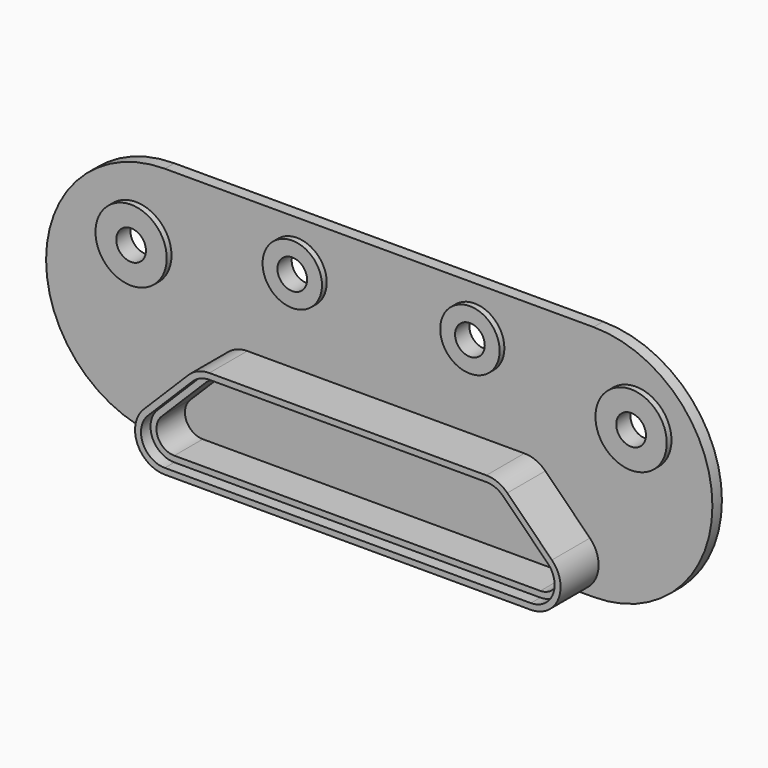
from build123d import *

# Parameters (mm, degrees)
F1_DEPTH  = 2
F3_DEPTH  = 8
F5_DEPTH  = 2
F7_DEPTH  = 6
F8_R      = 5
F8_R_2    = 6
F9_DEPTH  = 1
F10_R     = 2.5
F11_R     = 2.5
F12_DEPTH = 3.001


# Not quite as in the source:
# - a feature names something its author has since deleted; it is built from what else it names


with BuildPart() as f1:
    # F0 (on Front) → F1 (new body)
    with BuildSketch(Plane.XZ):
        with BuildLine():
            Line((-37.1916021632, -20), (34.9713978368, -20))
            ThreePointArc((34.9713978368, -20), (54.9713978368, 0), (34.9713978368, 20))
            Line((34.9713978368, 20), (-37.1916021632, 20))
            ThreePointArc((-37.1916021632, 20), (-57.1916021632, 0), (-37.1916021632, -20))
        make_face()
    extrude(amount=F1_DEPTH)

    # F2 (on face) → F3 (join)
    with BuildSketch(Plane.XZ.offset(2)):
        with BuildLine():
            Line((23.3145, -2.5), (0, -2.5))
            Line((0, -2.5), (-23.3145, -2.5))
            ThreePointArc((-23.3145, -2.5), (-25.2279171618, -2.8806023374), (-26.8500339059, -3.9644660941))
            Line((-26.8500339059, -3.9644660941), (-34.3500339059, -11.4644660941))
            ThreePointArc((-34.3500339059, -11.4644660941), (-35.4338976626, -16.9134171618), (-30.8145, -20))
            Line((-30.8145, -20), (0, -20))
            Line((0, -20), (30.8145, -20))
            ThreePointArc((30.8145, -20), (35.4338976626, -16.9134171618), (34.3500339059, -11.4644660941))
            Line((34.3500339059, -11.4644660941), (26.8500339059, -3.9644660941))
            ThreePointArc((26.8500339059, -3.9644660941), (25.2279171618, -2.8806023374), (23.3145, -2.5))
        make_face()
    extrude(amount=F3_DEPTH)

    # F4 (on face) → F5 (cut)
    with BuildSketch(Plane.XZ.offset(10)):
        with BuildLine():
            Line((-26.1429271247, -4.6715728753), (-33.6429271247, -12.1715728753))
            ThreePointArc((-33.6429271247, -12.1715728753), (-34.51001813, -16.5307337295), (-30.8145, -19))
            Line((-30.8145, -19), (30.8145, -19))
            ThreePointArc((30.8145, -19), (34.51001813, -16.5307337295), (33.6429271247, -12.1715728753))
            Line((33.6429271247, -12.1715728753), (26.1429271247, -4.6715728753))
            ThreePointArc((26.1429271247, -4.6715728753), (24.8452337295, -3.80448187), (23.3145, -3.5))
            Line((23.3145, -3.5), (-23.3145, -3.5))
            ThreePointArc((-23.3145, -3.5), (-24.8452337295, -3.80448187), (-26.1429271247, -4.6715728753))
        make_face()
    extrude(amount=-F5_DEPTH, mode=Mode.SUBTRACT)

    # F6 (on face) → F7 (cut)
    with BuildSketch(Plane.XZ.offset(8)):
        with BuildLine():
            ThreePointArc((30.8145, -18), (33.5861385975, -16.1480502971), (32.9358203436, -12.8786796564))
            Line((32.9358203436, -12.8786796564), (25.4358203436, -5.3786796564))
            ThreePointArc((25.4358203436, -5.3786796564), (24.4625502971, -4.7283614025), (23.3145, -4.5))
            Line((23.3145, -4.5), (-23.3145, -4.5))
            ThreePointArc((-23.3145, -4.5), (-24.4625502971, -4.7283614025), (-25.4358203436, -5.3786796564))
            Line((-25.4358203436, -5.3786796564), (-32.9358203436, -12.8786796564))
            ThreePointArc((-32.9358203436, -12.8786796564), (-33.5861385975, -16.1480502971), (-30.8145, -18))
            Line((-30.8145, -18), (30.8145, -18))
        make_face()
    extrude(amount=-F7_DEPTH, mode=Mode.SUBTRACT)

    # F8 (on face) → F9 (join)
    with BuildSketch(Plane.XZ.offset(2)):
        with Locations((-14.952, 12)):
            Circle(F8_R)
        with Locations((-42.0815, 7.5)):
            Circle(F8_R_2)
        with Locations((14.952, 12)):
            Circle(F8_R)
        with Locations((42.0815, 7.5)):
            Circle(F8_R_2)
    extrude(amount=F9_DEPTH)

    # F10 (on face) + F11 (on face) → F12 (cut, through all)
    with BuildSketch(Plane.XZ.offset(3)):
        with Locations((-14.952, 12)):
            Circle(F10_R)
        with Locations((14.952, 12)):
            Circle(F10_R)
    with BuildSketch(Plane.XZ.offset(3)):
        with Locations((-42.0815, 7.5)):
            Circle(F11_R)
        with Locations((42.0815, 7.5)):
            Circle(F11_R)
    extrude(amount=-F12_DEPTH, mode=Mode.SUBTRACT)


solid = f1.part
